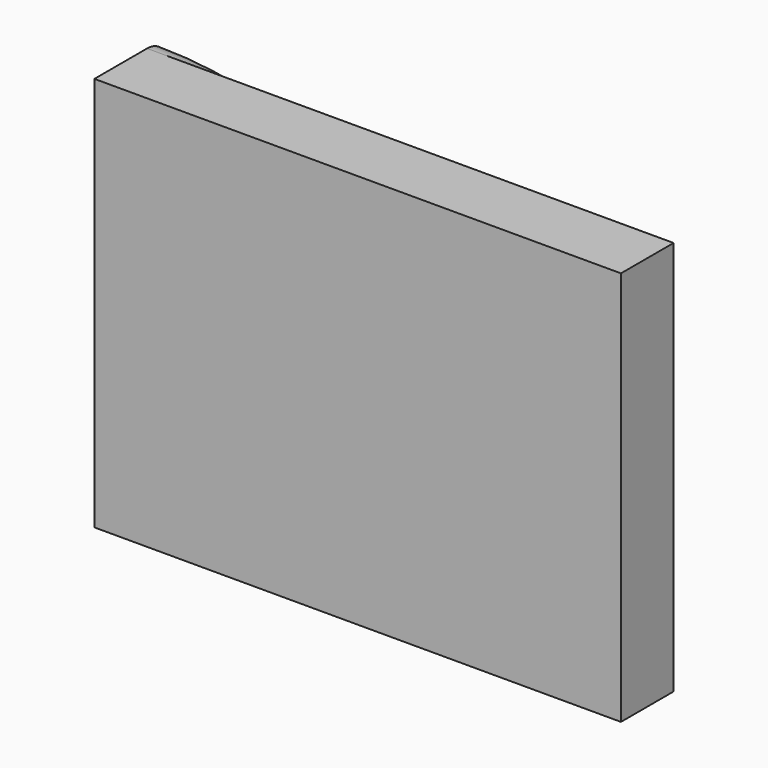
from build123d import *

# Parameters (mm, degrees)
F0_W     = 101.6
F0_H     = 76.2
F1_DEPTH = 12.7
F5_R     = 5.07999


# Not quite as in the source:
# - a fillet or chamfer is up to 0.001 mm smaller than in the source, because OpenCascade refuses the exact size


with BuildPart() as f1:
    # F0 (on Front) → F1 (new body)
    with BuildSketch(Plane.XZ):
        with Locations((50.8, 38.1)):
            Rectangle(F0_W, F0_H)
    extrude(amount=F1_DEPTH)


with BuildPart() as f4:
    # F4: sweep along a path in F3
    with BuildLine(Plane.XY) as f4_path:
        Line((13.2644446979, 0), (13.2644446979, 5.08))
    # F2 (on Front) → F4 (sweep)
    with BuildSketch(Plane.XZ):
        with BuildLine():
            ThreePointArc((0, 66.04), (46.6973318296, 46.6973318296), (66.04, 0))
            Line((66.04, 0), (76.2, 0))
            ThreePointArc((76.2, 0), (53.8815367264, 53.8815367264), (0, 76.2))
            Line((0, 76.2), (0, 66.04))
        make_face()
    sweep(path=f4_path.line)

    # F5 (radius 5.08 in the source; OpenCascade refuses exactly that, so slightly less here)
    f5_edges = [f4.edges().sort_by_distance(p)[0] for p in [
        (46.697332, 5.08, 46.697332),
        (53.881537, 5.08, 53.881537),
    ]]
    fillet(f5_edges, radius=F5_R)


solid = Compound([f1.part, f4.part])
